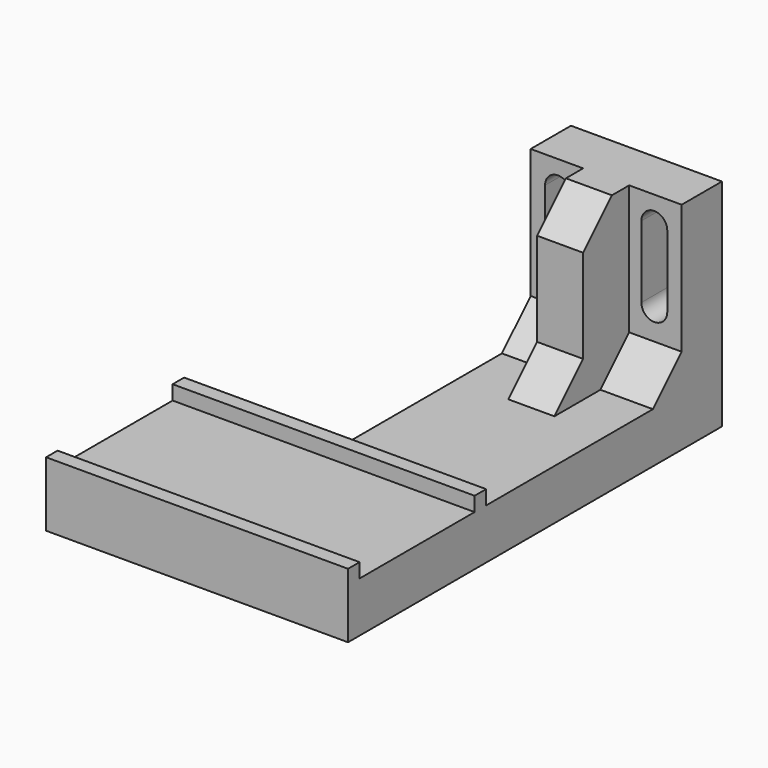
from build123d import *

# Parameters (mm, degrees)
F1_DEPTH = 10.5
F3_DEPTH = 25
F2_W     = 3.2
F2_H     = 23
F4_DEPTH = 15
F5_SIZE  = 5
F8_DEPTH = 21


with BuildPart() as f1:
    # F0 (on Right) → F1 (new body)
    with BuildSketch(Plane.YZ):
        Polygon((0, 0), (0, -23), (-46.5, -23), (-51, -23), (-58, -23), (-58, -30), (7, -30), (7, 0), align=None)
    extrude(amount=F1_DEPTH)

    # F2 (on face) → F3 (cut)
    with BuildSketch(Plane(origin=(0, 7, 0), x_dir=(-1, 0, 0), z_dir=(0, 1, 0))):
        with BuildLine():
            Line((-4.9, -13.8), (-4.9, -3.8))
            ThreePointArc((-4.9, -3.8), (-6.7, -2), (-8.5, -3.8))
            Line((-8.5, -3.8), (-8.5, -13.8))
            ThreePointArc((-8.5, -13.8), (-6.7, -15.6), (-4.9, -13.8))
        make_face()
    extrude(amount=-F3_DEPTH, mode=Mode.SUBTRACT)

    # F2 (on face) → F4 (join)
    with BuildSketch(Plane(origin=(0, 7, 0), x_dir=(-1, 0, 0), z_dir=(0, 1, 0))):
        with Locations((-1.6, -11.5)):
            Rectangle(F2_W, F2_H)
    extrude(amount=-F4_DEPTH)

    # F5
    f5_edges = [f1.edges().sort_by_distance(p)[0] for p in [
        (1.6, -8, -23),
        (1.6, -8, 0),
        (6.85, 0, -23),
    ]]
    chamfer(f5_edges, length=F5_SIZE)

    # F6: F1 across face


with BuildPart() as f1_1:
    add(f1.part)
    add(f1.part.mirror(Plane(origin=(0, -14.7708333333, -20.3385416667), x_dir=(0, -1, 0), z_dir=(-1, 0, 0))))

    # F7 (on face) → F8 (join, symmetric)
    with BuildSketch(Plane(origin=(-10.5, 0, 0), x_dir=(0, -1, 0), z_dir=(-1, 0, 0))):
        Polygon((34, -30), (58, -30), (58, -21), (56, -21), (56, -23), (36, -23), (36, -21), (34, -21), align=None)
    extrude(amount=F8_DEPTH, both=True)


solid = f1_1.part
